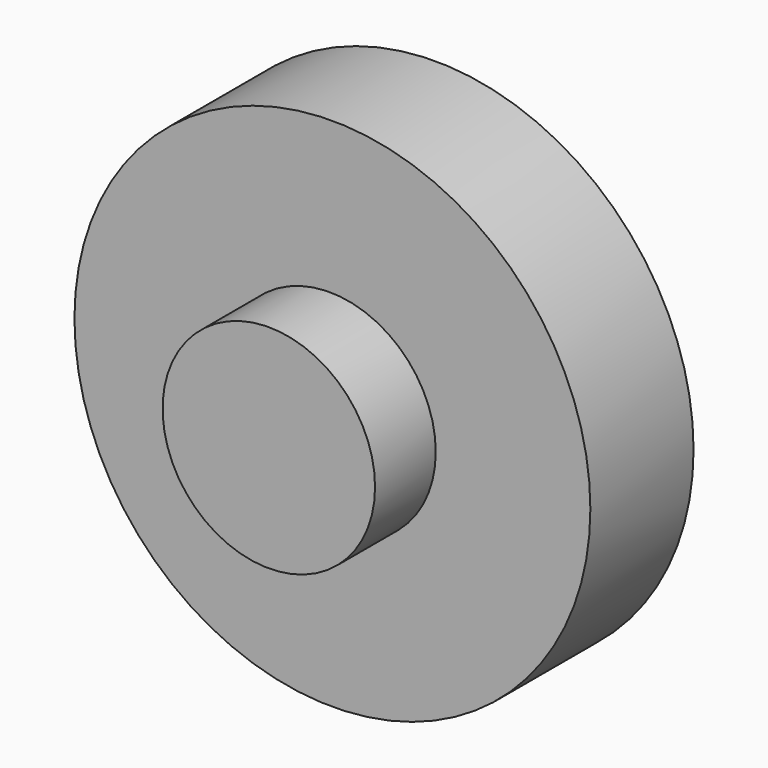
from build123d import *

# Parameters (mm, degrees)
F0_R     = 170
F1_DEPTH = 85
F2_R     = 70
F3_DEPTH = 50


# Not quite as in the source:
# - the program builds the solid bodies; features that only make, move or delete a surface that nothing else refers to are left out


with BuildPart() as f1:
    # F0 (on Front) → F1 (new body)
    with BuildSketch(Plane.XZ):
        Circle(F0_R)
    extrude(amount=F1_DEPTH)

    # F2 (on face) → F3 (join)
    with BuildSketch(Plane.XZ.offset(85)):
        with Locations((-1.8989939419, 0)):
            Circle(F2_R)
    extrude(amount=F3_DEPTH)


solid = f1.part
